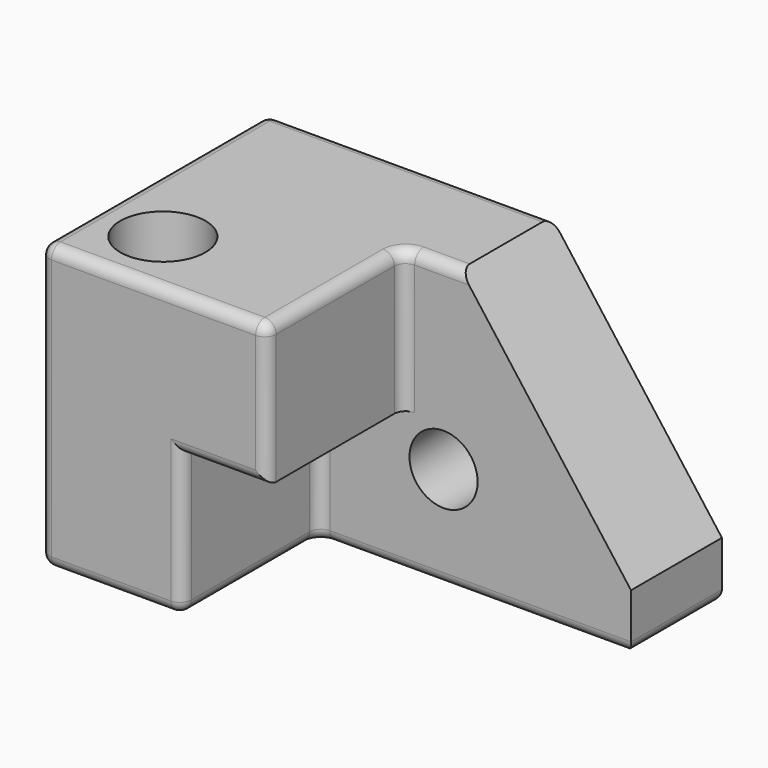
from build123d import *

# Parameters (mm, degrees)
F0_W     = 203.2
F0_H     = 127
F1_DEPTH = 127
F3_DEPTH = 76.2
F4_SIZE2 = 101.6
F4_SIZE  = 76.2
F5_R     = 5.08
F6_R     = 15.24
F7_DEPTH = 50.8
F8_R     = 19.05
F9_DEPTH = 127


with BuildPart() as f1:
    # F0 (on Front) → F1 (new body)
    with BuildSketch(Plane.XZ):
        with Locations((0.1851254753, -0.3465637565)):
            Rectangle(F0_W, F0_H)
    extrude(amount=F1_DEPTH)

    # F2 (on face) → F3 (cut)
    with BuildSketch(Plane.XZ.offset(127)):
        Polygon((101.7851254753, 63.1534362435), (0, 63.1534362435), (0, 0), (-37.9148745247, 0), (-37.9148745247, -63.8465637565), (101.7851254753, -63.8465637565), align=None)
    extrude(amount=-F3_DEPTH, mode=Mode.SUBTRACT)

    # F4
    f4_edges = [f1.edges().sort_by_distance(p)[0] for p in [
        (101.785125, -25.4, 63.153436),
    ]]
    f4_side = f1.faces().sort_by_distance((-21.603245, -52.585928, 63.153436))[0]
    chamfer(f4_edges, length=F4_SIZE, length2=F4_SIZE2, reference=f4_side)

    # F5
    f5_edges = [f1.edges().sort_by_distance(p)[0] for p in [
        (-50.707437, -127, 63.153436),
        (0, -88.9, 63.153436),
        (0, -127, 31.576718),
        (-18.957437, -127, 0),
        (-37.914875, -127, -31.923282),
        (-37.914875, -50.8, -31.923282),
        (12.792563, -50.8, 63.153436),
        (0, -50.8, 31.576718),
        (-37.914875, 0, 63.153436),
        (-101.414875, -63.5, 63.153436),
        (-101.414875, -127, -0.346564),
        (-101.414875, 0, -0.346564),
        (-69.664875, -127, -63.846564),
        (-37.914875, -88.9, -63.846564),
        (101.785125, -25.4, -63.846564),
        (0.185125, 0, -63.846564),
        (-101.414875, -63.5, -63.846564),
        (31.935125, -50.8, -63.846564),
    ]]
    fillet(f5_edges, radius=F5_R)

    # F6 (on face) → F7 (cut, through all)
    with BuildSketch(Plane.XZ.offset(50.8)):
        with Locations((17.9651254753, -18.1265637565)):
            Circle(F6_R)
    extrude(amount=-F7_DEPTH, mode=Mode.SUBTRACT)

    # F8 (on face) → F9 (cut, through all)
    with BuildSketch(Plane.XY.offset(63.1534362435)):
        with Locations((-70.9348745247, -96.52)):
            Circle(F8_R)
    extrude(amount=-F9_DEPTH, mode=Mode.SUBTRACT)


solid = f1.part
